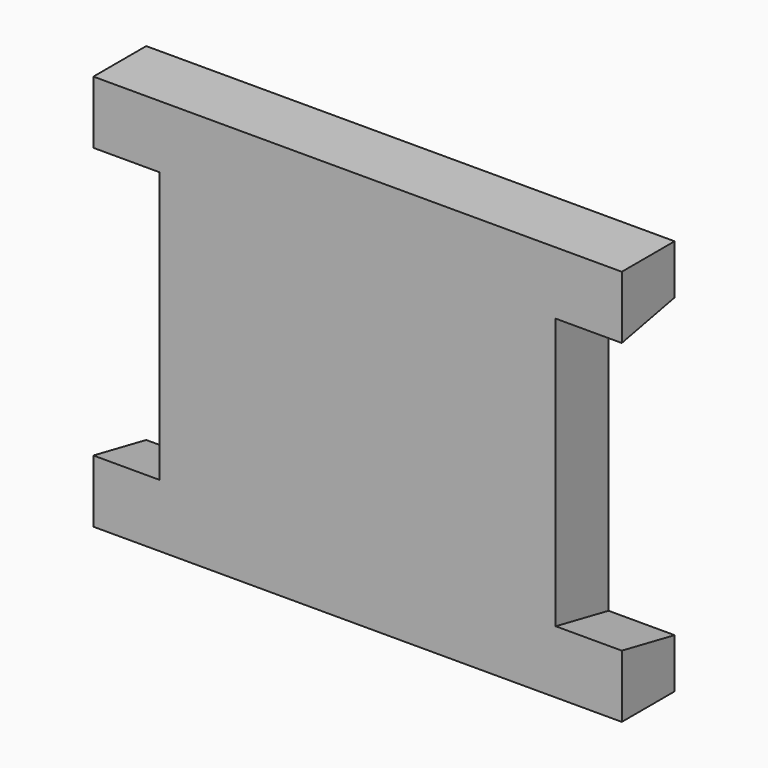
from build123d import *

# Parameters (mm, degrees)
F0_W     = 12.7
F0_H     = 76.2
F1_DEPTH = 50.8
F3_DEPTH = 12.7


# Not quite as in the source:
# - a pattern or mirror of a feature is missing from the dataset's text; its kind, count and spacing are read off the source's solid


with BuildPart() as f1:
    # F0 (on Right) → F1 (new body, symmetric)
    with BuildSketch(Plane.YZ):
        Rectangle(F0_W, F0_H)
    extrude(amount=F1_DEPTH, both=True)

    # F2 (on face) → F3 (cut)
    with BuildSketch(Plane(origin=(-50.8, 0, 0), x_dir=(0, -1, 0), z_dir=(-1, 0, 0))):
        Polygon((6.35, -26.0372895852), (6.35, 26.0372895852), (-6.35, 28.575), (-6.35, -28.575), align=None)
    f3 = extrude(amount=-F3_DEPTH, mode=Mode.SUBTRACT)

    # F3_copies: F3 across plane
    add(f3.mirror(Plane(origin=(0, 0, 0), x_dir=(0, 0, 1), z_dir=(1, 0, 0))), mode=Mode.SUBTRACT)


solid = f1.part
